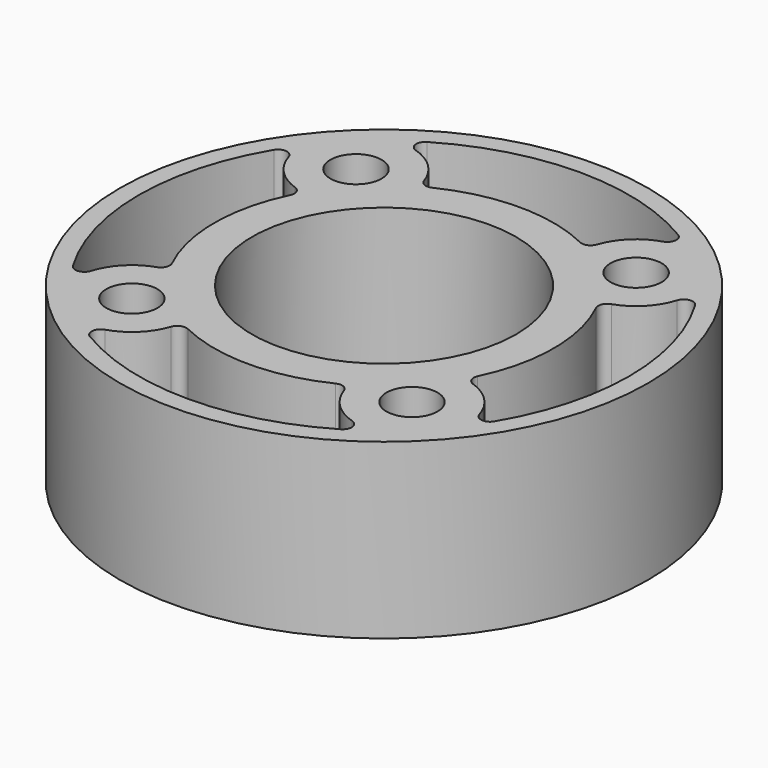
from build123d import *

# Parameters (mm, degrees)
F0_R            = 22.225
F0_R_2          = 2.15265
F0_R_3          = 11.1125
F1_DEPTH        = 14.5749645
F3_DEPTH        = 14.5749645
F3_COPIES_COUNT = 4
F4_R            = 0.762


# Not quite as in the source:
# - a pattern or mirror of a feature is missing from the dataset's text; its kind, count and spacing are read off the source's solid


with BuildPart() as f1:
    # F0 (on Top) → F1 (new body)
    with BuildSketch(Plane.XY):
        Circle(F0_R)
        with Locations((-11.7865861589, -11.7865861589)):
            Circle(F0_R_2, mode=Mode.SUBTRACT)
        with Locations((11.7865861589, -11.7865861589)):
            Circle(F0_R_2, mode=Mode.SUBTRACT)
        with Locations((-11.7865861589, 11.7865861589)):
            Circle(F0_R_2, mode=Mode.SUBTRACT)
        Circle(F0_R_3, mode=Mode.SUBTRACT)
        with Locations((11.7865861589, 11.7865861589)):
            Circle(F0_R_2, mode=Mode.SUBTRACT)
    extrude(amount=F1_DEPTH)

    # F2 (on face) → F3 (cut, through all)
    with BuildSketch(Plane.XY.offset(14.5749645)):
        with BuildLine():
            ThreePointArc((12.3798449874, -16.511990926), (8.879869507, -15.5591720831), (7.0661070567, -12.4178414917))
            ThreePointArc((7.0661070567, -12.4178414917), (0, -14.2875), (-7.0661070567, -12.4178414917))
            ThreePointArc((-7.0661070567, -12.4178414917), (-8.879869507, -15.5591720831), (-12.3798449874, -16.511990926))
            ThreePointArc((-12.3798449874, -16.511990926), (0, -20.6375), (12.3798449874, -16.511990926))
        make_face()
    f3 = extrude(amount=-F3_DEPTH, mode=Mode.SUBTRACT)

    # F3_copies: F3 ×4 about axis
    f3_copies_axis = Axis((0, 0, 0), (0, 0, 1))
    for i in range(1, F3_COPIES_COUNT):
        add(f3.rotate(f3_copies_axis, i * 360 / F3_COPIES_COUNT), mode=Mode.SUBTRACT)

    # F4
    f4_edges = [f1.edges().sort_by_distance(p)[0] for p in [
        (7.066107, -12.417841, 7.287482),
        (12.379845, -16.511991, 7.287482),
        (-7.066107, -12.417841, 7.287482),
        (-12.379845, -16.511991, 7.287482),
        (12.417841, -7.066107, 7.287482),
        (16.511991, -12.379845, 7.287482),
        (12.417841, 7.066107, 7.287482),
        (16.511991, 12.379845, 7.287482),
        (-12.417841, 7.066107, 7.287482),
        (-16.511991, 12.379845, 7.287482),
        (-16.511991, -12.379845, 7.287482),
        (-12.417841, -7.066107, 7.287482),
        (7.066107, 12.417841, 7.287482),
        (12.379845, 16.511991, 7.287482),
        (-7.066107, 12.417841, 7.287482),
        (-12.379845, 16.511991, 7.287482),
    ]]
    fillet(f4_edges, radius=F4_R)


solid = f1.part
